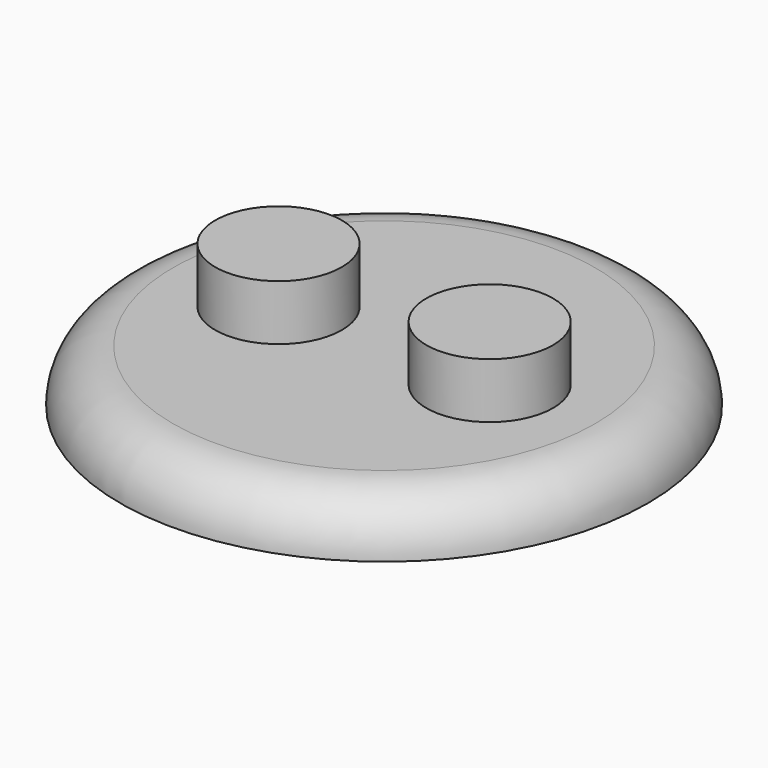
from build123d import *

# Parameters (mm, degrees)
F0_R     = 10
F1_DEPTH = 2
F2_R     = 1.99999
F3_R     = 2.4
F4_DEPTH = 2.1


# Not quite as in the source:
# - a fillet or chamfer is up to 0.001 mm smaller than in the source, because OpenCascade refuses the exact size


with BuildPart() as f1:
    # F0 (on Top) → F1 (new body)
    with BuildSketch(Plane.XY):
        Circle(F0_R)
    extrude(amount=F1_DEPTH)

    # F2 (radius 2 in the source; OpenCascade refuses exactly that, so slightly less here)
    f2_edges = [f1.edges().sort_by_distance(p)[0] for p in [
        (-10, 0, 2),
    ]]
    fillet(f2_edges, radius=F2_R)

    # F3 (on face) → F4 (join)
    with BuildSketch(Plane.XY.offset(2)):
        with Locations((-4, 0)):
            Circle(F3_R)
        with Locations((4, 0)):
            Circle(F3_R)
    extrude(amount=F4_DEPTH)


solid = f1.part
